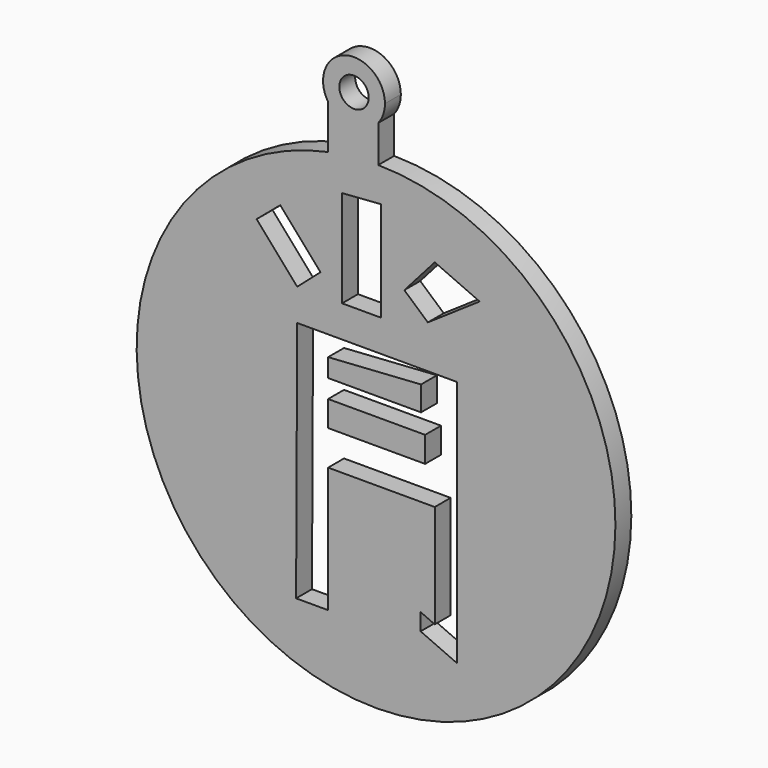
from build123d import *

# Parameters (mm, degrees)
F0_R     = 2.3475480715
F1_DEPTH = 3.175
F3_DEPTH = 3.175


# Not quite as in the source:
# - a feature names something its author has since deleted; it is built from what else it names


with BuildPart() as f1:
    # F0 (on Front) → F1 (new body)
    with BuildSketch(Plane.XZ):
        with BuildLine():
            ThreePointArc((31.7726456889, 74.1154716994), (15.2436424275, 7.0166806556), (77.6749893029, 36.6440773635))
            ThreePointArc((77.6749893029, 36.6440773635), (66.5982509819, 63.5621034518), (39.7841440278, 74.8880881142))
            ThreePointArc((39.7841440278, 74.8880881142), (35.7580139785, 74.7131155477), (31.7726456889, 74.1154716994))
        make_face()
        with BuildLine():
            ThreePointArc((31.7726456889, 74.1154716994), (35.7580139785, 74.7131155477), (39.7841440278, 74.8880881142))
            Line((39.7841440278, 74.8880881142), (39.7841440278, 80.807211974))
            ThreePointArc((39.7841440278, 80.807211974), (35.6867088214, 78.9353641119), (31.7726456889, 81.1653639963))
            Line((31.7726456889, 81.1653639963), (31.7726456889, 74.1154716994))
        make_face()
        with BuildLine():
            ThreePointArc((31.7726456889, 81.1653639963), (35.6867088214, 78.9353641119), (39.7841440278, 80.807211974))
            ThreePointArc((39.7841440278, 80.807211974), (40.5757369766, 82.2500098688), (40.8497276092, 83.8727280498))
            ThreePointArc((40.8497276092, 83.8727280498), (34.4948204969, 88.6088455606), (31.7726456889, 81.1653639963))
        make_face()
        with Locations((35.9074324369, 83.8727280498)):
            Circle(F0_R, mode=Mode.SUBTRACT)
    extrude(amount=F1_DEPTH)

    # F2 (on face) → F3 (cut)
    with BuildSketch(Plane.XZ.offset(3.175)):
        Polygon((24.1258461707, 64.1513620911), (20.3500986099, 60.9632693231), (26.828661561, 53.5591952503), (30.5470783074, 56.8128089679), align=None)
        Polygon((40.2485467494, 69.5242285728), (34.0013615787, 69.061473012), (34.0013615787, 53.5591952503), (40.2485467494, 53.5591952503), align=None)
        Polygon((55.9822022915, 60.9632693231), (48.8095022738, 64.1513620911), (43.9505800605, 58.649495244), (47.7068929317, 55.3321426876), align=None)
        Polygon((52.3958522826, 48.4688952565), (26.828661561, 48.4688952565), (26.6563948244, 9.6785360947), (31.7726456889, 9.6785360947), (31.7726456889, 29.7273341566), (48.8095022738, 29.7273341566), (48.8095022738, 13.2189297204), (46.5458819901, 14.2250545323), (46.5458819901, 11.503547954), (52.3958522826, 8.9033767581), align=None)
        Polygon((34.3574807048, 35.2874398232), (31.7726456889, 35.2874398232), (31.7726456889, 39.3776521087), (47.2710616887, 39.3776521087), (47.2710616887, 35.2874398232), (36.1486673355, 35.2874398232), align=None, mode=Mode.SUBTRACT)
        Polygon((31.7726456889, 42.3226058483), (31.7726456889, 45.2675558627), (46.6166287661, 46.2492071092), (46.6166287661, 42.3226058483), align=None, mode=Mode.SUBTRACT)
    extrude(amount=-F3_DEPTH, mode=Mode.SUBTRACT)


solid = f1.part
